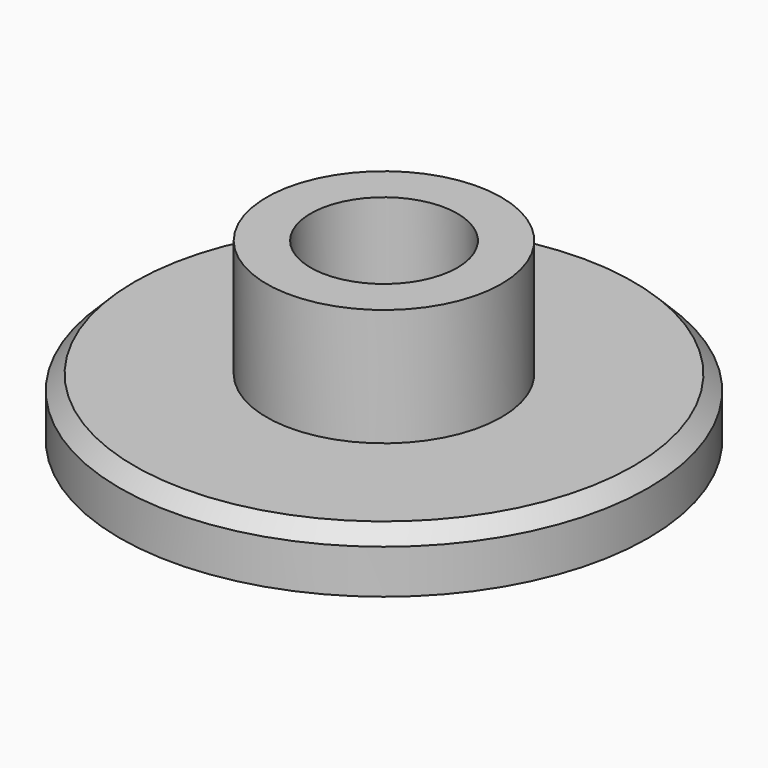
from build123d import *

# Parameters (mm, degrees)
F0_R     = 9
F1_DEPTH = 2
F2_R     = 4
F3_DEPTH = 4
F4_R     = 2.5
F5_DEPTH = 3
F6_SIZE  = 0.5


with BuildPart() as f1:
    # F0 (on Top) → F1 (new body)
    with BuildSketch(Plane.XY):
        Circle(F0_R)
    extrude(amount=F1_DEPTH)

    # F2 (on face) → F3 (join)
    with BuildSketch(Plane.XY.offset(2)):
        Circle(F2_R)
    extrude(amount=F3_DEPTH)

    # F4 (on face) → F5 (cut)
    with BuildSketch(Plane.XY.offset(6)):
        Circle(F4_R)
    extrude(amount=-F5_DEPTH, mode=Mode.SUBTRACT)

    # F6
    f6_edges = [f1.edges().sort_by_distance(p)[0] for p in [
        (-9, 0, 2),
    ]]
    chamfer(f6_edges, length=F6_SIZE)


solid = f1.part
